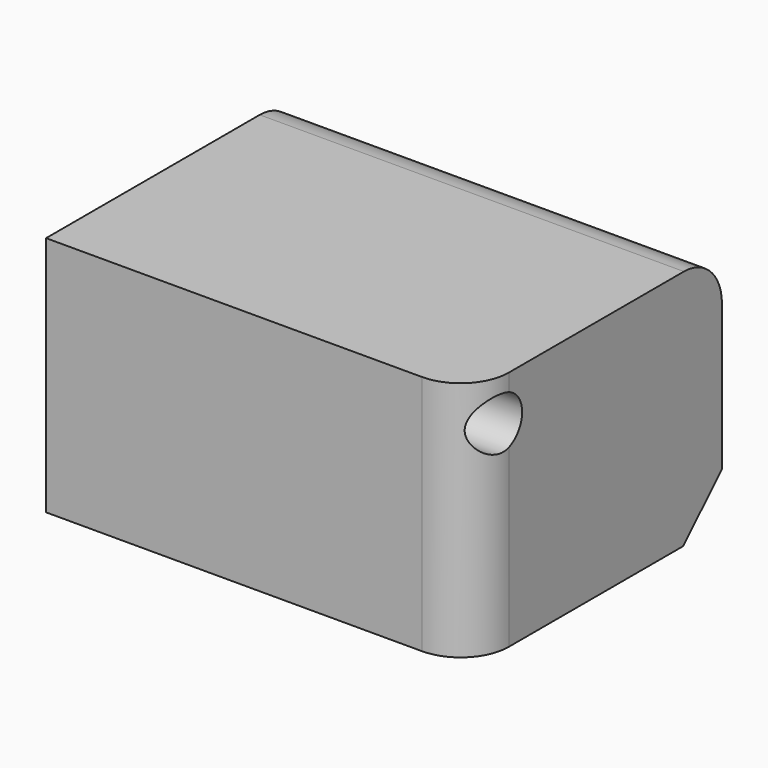
from build123d import *

# Parameters (mm, degrees)
F0_W        = 44.6331575513
F0_H        = 33.0944694579
F1_DEPTH    = 25.4
F2_R        = 5
F3_SIZE     = 5.08
F4_R        = 2.7454645763
F5_DEPTH    = 25.4
F6_T1_DEPTH = 50.8


# Not quite as in the source:
# - a fillet or chamfer that OpenCascade refuses, or shapes differently, is made with other operations: its cross-section is extruded or revolved along the edge and cut away or added


with BuildPart() as f1:
    # F0 (on Top) → F1 (new body)
    with BuildSketch(Plane.XY):
        with Locations((22.3165787756, -16.5472347289)):
            Rectangle(F0_W, F0_H)
    extrude(amount=F1_DEPTH)

    # F2
    f2_edges = [f1.edges().sort_by_distance(p)[0] for p in [
        (22.316579, 0, 25.4),
    ]]
    fillet(f2_edges, radius=F2_R)

    # F3
    f3_edges = [f1.edges().sort_by_distance(p)[0] for p in [
        (22.316579, 0, 0),
    ]]
    chamfer(f3_edges, length=F3_SIZE)

    # F4 (on face) → F5 (cut)
    with BuildSketch(Plane.YZ.offset(44.6331575513)):
        with Locations((-29.0195755661, 21.0298281163)):
            Circle(F4_R)
    extrude(amount=-F5_DEPTH, mode=Mode.SUBTRACT)

    # F6: fillet of radius 5.08 on 1 edges, made by hand

    # F6_s2 → F6_t1 (cut)
    with BuildSketch(Plane.XY.offset(-12.7)):
        with BuildLine():
            ThreePointArc((44.6331575513, -28.0144694579), (43.1452599997, -31.6065719063), (39.5531575513, -33.0944694579))
            Line((39.5531575513, -33.0944694579), (44.6331575513, -33.0944694579))
            Line((44.6331575513, -33.0944694579), (44.6331575513, -28.0144694579))
        make_face()
    extrude(amount=F6_T1_DEPTH, mode=Mode.SUBTRACT)


solid = f1.part
